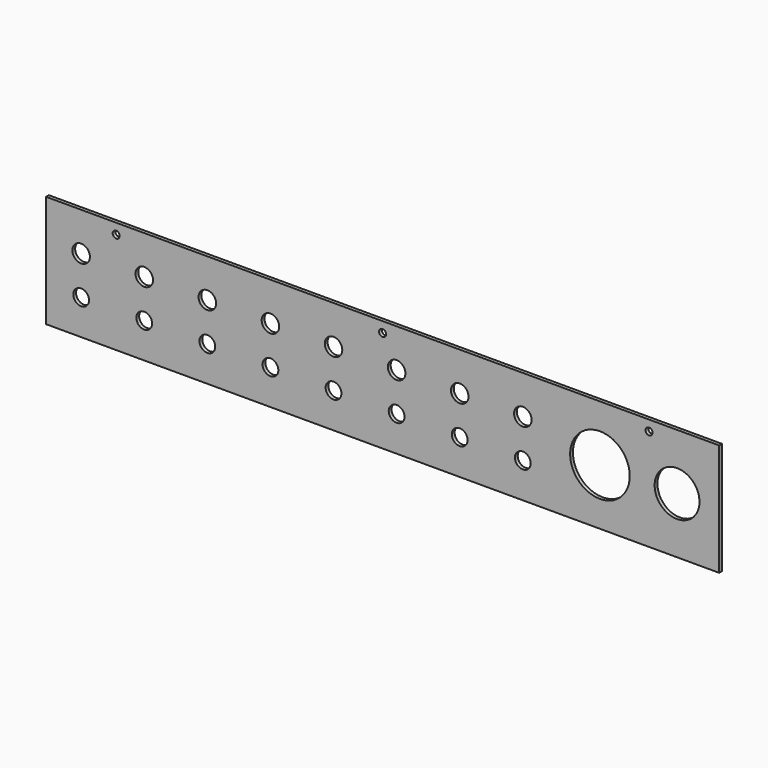
from build123d import *

# Parameters (mm, degrees)
F0_W      = 609.6
F0_H      = 101.6
F1_DEPTH  = 3.175
F2_R      = 7.14375
F3_DEPTH  = 3.176
F4_R      = 26.9875
F5_DEPTH  = 3.176
F6_R      = 20.32
F7_DEPTH  = 3.176
F8_R      = 7.9375
F9_DEPTH  = 3.176
F10_R     = 3.175
F11_DEPTH = 3.176


# Not quite as in the source:
# - a feature names something its author has since deleted; it is built from what else it names


with BuildPart() as f1:
    # F0 (on Front) → F1 (new body)
    with BuildSketch(Plane.XZ):
        with Locations((304.8, 50.8)):
            Rectangle(F0_W, F0_H)
    extrude(amount=F1_DEPTH)

    # F2 (on face) → F3 (cut, through all)
    with BuildSketch(Plane.XZ.offset(3.175)):
        with Locations((31.75, 31.75)):
            Circle(F2_R)
        with Locations((88.9, 31.75)):
            Circle(F2_R)
        with Locations((146.05, 31.75)):
            Circle(F2_R)
        with Locations((203.2, 31.75)):
            Circle(F2_R)
        with Locations((260.35, 31.75)):
            Circle(F2_R)
        with Locations((317.5, 31.75)):
            Circle(F2_R)
        with Locations((374.65, 31.75)):
            Circle(F2_R)
        with Locations((431.8, 31.75)):
            Circle(F2_R)
    extrude(amount=-F3_DEPTH, mode=Mode.SUBTRACT)

    # F4 (on face) → F5 (cut, through all)
    with BuildSketch(Plane.XZ.offset(3.175)):
        with Locations((501.65, 50.8)):
            Circle(F4_R)
    extrude(amount=-F5_DEPTH, mode=Mode.SUBTRACT)

    # F6 (on face) → F7 (cut, through all)
    with BuildSketch(Plane.XZ.offset(3.175)):
        with Locations((571.5, 50.8)):
            Circle(F6_R)
    extrude(amount=-F7_DEPTH, mode=Mode.SUBTRACT)

    # F8 (on face) → F9 (cut, through all)
    with BuildSketch(Plane.XZ.offset(3.175)):
        with Locations((31.75, 66.675)):
            Circle(F8_R)
        with Locations((88.9, 66.675)):
            Circle(F8_R)
        with Locations((146.05, 66.675)):
            Circle(F8_R)
        with Locations((203.2, 66.675)):
            Circle(F8_R)
        with Locations((260.35, 66.675)):
            Circle(F8_R)
        with Locations((317.5, 66.675)):
            Circle(F8_R)
        with Locations((374.65, 66.675)):
            Circle(F8_R)
        with Locations((431.8, 66.675)):
            Circle(F8_R)
    extrude(amount=-F9_DEPTH, mode=Mode.SUBTRACT)

    # F10 (on face) → F11 (cut, through all)
    with BuildSketch(Plane.XZ.offset(3.175)):
        with Locations((63.5, 92.075)):
            Circle(F10_R)
        with Locations((304.8, 92.075)):
            Circle(F10_R)
        with Locations((546.1, 92.075)):
            Circle(F10_R)
    extrude(amount=-F11_DEPTH, mode=Mode.SUBTRACT)


solid = f1.part
